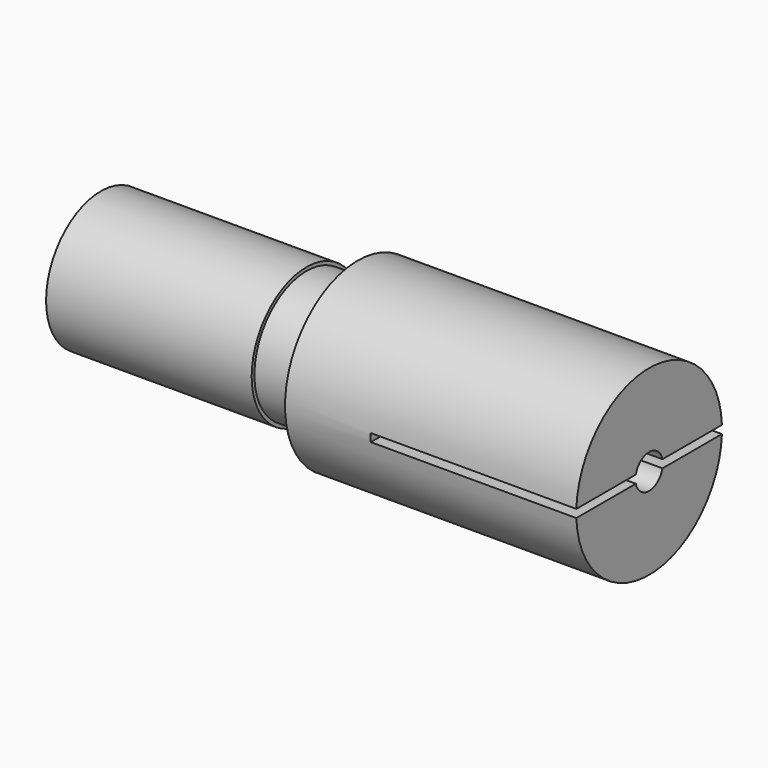
from build123d import *

# Parameters (mm, degrees)
F0_R     = 12.065
F1_DEPTH = 9.525
F2_R     = 16.8783
F2_R_2   = 12.065
F3_DEPTH = 53.975
F4_R     = 12.7
F4_R_2   = 12.065
F5_DEPTH = 38.1
F6_R     = 3.175
F7_DEPTH = 25.4
F9_DEPTH = 38.1


with BuildPart() as f1:
    # F0 (on Right) → F1 (new body)
    with BuildSketch(Plane.YZ):
        Circle(F0_R)
    extrude(amount=F1_DEPTH)

    # F2 (on face) → F3 (join)
    with BuildSketch(Plane.YZ.offset(9.525)):
        Circle(F2_R)
        Circle(F2_R_2, mode=Mode.SUBTRACT)
        Circle(F2_R_2)
    extrude(amount=F3_DEPTH)

    # F4 (on face) → F5 (join)
    with BuildSketch(Plane(origin=(0, 0, 0), x_dir=(0, -1, 0), z_dir=(-1, 0, 0))):
        Circle(F4_R)
        Circle(F4_R_2, mode=Mode.SUBTRACT)
        Circle(F4_R_2)
    extrude(amount=F5_DEPTH)

    # F6 (on face) → F7 (cut)
    with BuildSketch(Plane.YZ.offset(63.5)):
        Circle(F6_R)
    extrude(amount=-F7_DEPTH, mode=Mode.SUBTRACT)

    # F8 (on face) → F9 (cut)
    with BuildSketch(Plane.YZ.offset(63.5)):
        with BuildLine():
            ThreePointArc((-16.8618667917, 0.7446201635), (-16.8783, 0), (-16.8618667917, -0.7446201635))
            Line((-16.8618667917, -0.7446201635), (-3.086448738, -0.7446201635))
            ThreePointArc((-3.086448738, -0.7446201635), (-3.175, 0), (-3.086448738, 0.7446201635))
            Line((-3.086448738, 0.7446201635), (-16.8618667917, 0.7446201635))
        make_face()
        with BuildLine():
            Line((3.086448738, -0.7446201635), (16.8618667917, -0.7446201635))
            ThreePointArc((16.8618667917, -0.7446201635), (16.8741911978, -0.3724007378), (16.8783, 0))
            ThreePointArc((16.8783, 0), (16.8741911978, 0.3724007378), (16.8618667917, 0.7446201635))
            Line((16.8618667917, 0.7446201635), (3.086448738, 0.7446201635))
            ThreePointArc((3.086448738, 0.7446201635), (3.1527844632, 0.3749334987), (3.175, 0))
            ThreePointArc((3.175, 0), (3.1527844632, -0.3749334987), (3.086448738, -0.7446201635))
        make_face()
    extrude(amount=-F9_DEPTH, mode=Mode.SUBTRACT)


solid = f1.part
